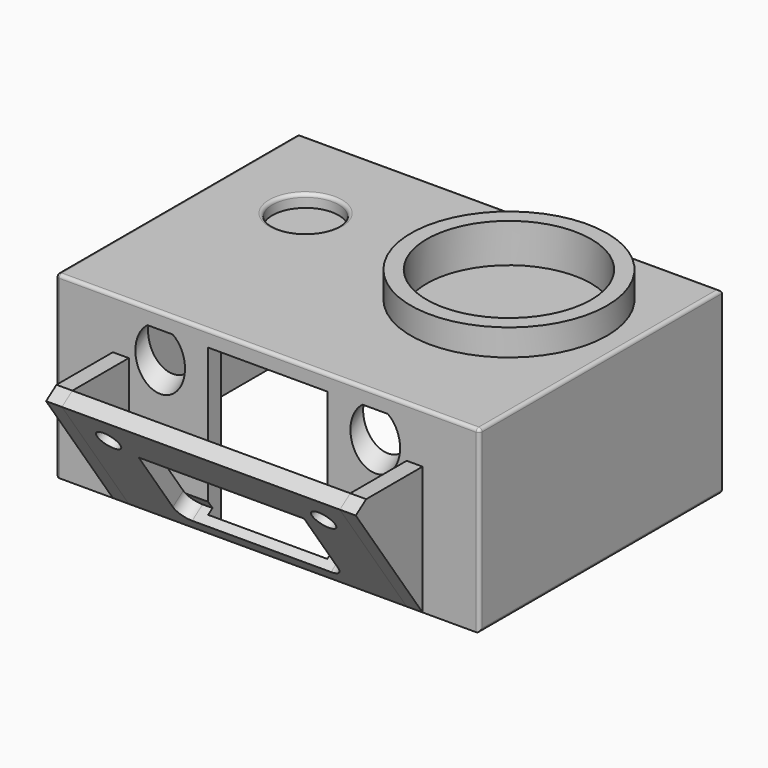
from build123d import *

# Parameters (mm, degrees)
F5_W         = 64
F5_H         = 45.8
F5_W_2       = 59.2
F5_H_2       = 41
F6_DEPTH     = 24.7
F7_W         = 64
F7_H         = 45.8
F7_W_2       = 59.2
F7_H_2       = 41
F8_DEPTH     = 2.4
F9_R         = 5
F10_DEPTH    = 1.9
F11_R        = 14.82
F11_R_2      = 12.42
F12_DEPTH    = 4
F13_DEPTH    = 1.9
F14_R        = 5
F15_DEPTH    = 2.4
F17_R        = 1.75
F18_DEPTH    = 2.4
F20_DEPTH    = 2.4
F22_DEPTH    = 2.4
F23_R        = 1.75
F24_REACH    = 60.3061382673
F25_R        = 0.5
F26_W        = 18
F26_H        = 2.4
F27_DEPTH    = 24.7
F28_R        = 3.75
F29_REACH    = 63.5629925168
F31_DEPTH    = 2.4
F32_T1_DEPTH = 2.4


# Not quite as in the source:
# - a fillet or chamfer that OpenCascade refuses, or shapes differently, is made with other operations: its cross-section is extruded or revolved along the edge and cut away or added
# - a feature names something its author has since deleted; it is built from what else it names


with BuildPart() as f6:
    # F5 (on Top) → F6 (new body)
    with BuildSketch(Plane.XY):
        Rectangle(F5_W, F5_H)
        Rectangle(F5_W_2, F5_H_2, mode=Mode.SUBTRACT)
    extrude(amount=F6_DEPTH)

    # F7 (on face) → F8 (join)
    with BuildSketch(Plane.XY.offset(24.7)):
        Rectangle(F7_W, F7_H)
        Rectangle(F7_W_2, F7_H_2, mode=Mode.SUBTRACT)
        Rectangle(F7_W_2, F7_H_2)
    extrude(amount=F8_DEPTH)

    # F9 (on face) → F10 (cut)
    with BuildSketch(Plane.XY.offset(27.1)):
        with Locations((-18.6, 7.5)):
            Circle(F9_R)
    extrude(amount=-F10_DEPTH, mode=Mode.SUBTRACT)

    # F11 (on face) → F12 (join)
    with BuildSketch(Plane.XY.offset(27.1)):
        with Locations((13.926, 5.264)):
            Circle(F11_R)
        with Locations((13.926, 5.264)):
            Circle(F11_R_2, mode=Mode.SUBTRACT)
    extrude(amount=F12_DEPTH)

    # F13 (cut): a face of the model
    f13_faces = [f6.faces().sort_by_distance(p)[0] for p in [
        (13.926, 5.264, 27.1),
    ]]
    extrude(f13_faces, amount=-F13_DEPTH, mode=Mode.SUBTRACT)

    # F14 (on face) → F15 (cut)
    with BuildSketch(Plane(origin=(0, 22.9, 0), x_dir=(-1, 0, 0), z_dir=(0, 1, 0))):
        with Locations((17.1, 13.55)):
            Circle(F14_R)
    extrude(amount=-F15_DEPTH, mode=Mode.SUBTRACT)

    # F17 (on face) → F18 (join)
    with BuildSketch(Plane(origin=(0, -15.3661306411, -10.759480508), x_dir=(-1, 0, 0), z_dir=(0, 0.8191520443, 0.5735764364))):
        Polygon((0, 24.1349003924), (0, 13.1349003924), (21, 13.1349003924), (21, 35.1349003924), (0, 35.1349003924), align=None)
        with Locations((16.25, 30.1349003924)):
            Circle(F17_R, mode=Mode.SUBTRACT)
        Polygon((-21, 13.1349003924), (0, 13.1349003924), (0, 24.1349003924), (0, 35.1349003924), (-21, 35.1349003924), align=None)
        with Locations((-16.25, 30.1349003924)):
            Circle(F17_R, mode=Mode.SUBTRACT)
    extrude(amount=F18_DEPTH)

    # F19 (on face) → F20 (join)
    with BuildSketch(Plane(origin=(-21, 0, 0), x_dir=(0, -1, 0), z_dir=(-1, 0, 0))):
        Polygon((22.9, 0), (35.5186815997, 18.0213449744), (33.5527166934, 19.3979284216), (22.9, 19.3979284216), align=None)
    extrude(amount=F20_DEPTH)

    # F21 (on face) → F22 (join)
    with BuildSketch(Plane.YZ.offset(21)):
        Polygon((-35.5186815997, 18.0213449744), (-22.9, 0), (-22.9, 19.3979284216), (-33.5527166934, 19.3979284216), align=None)
    extrude(amount=F22_DEPTH)

    f24_end = f6.faces().sort_by_distance((0, 0, 24.7))[0]
    # F23 (on face) → F24 (cut, up to a face of the model that its end follows)
    with BuildSketch(Plane(origin=(0, -15.3661306411, -10.759480508), x_dir=(1, 0, 0), z_dir=(0, -0.8191520443, -0.5735764364))):
        with Locations((-16.25, 30.1349003924)):
            Circle(F23_R)
        with Locations((16.25, 30.1349003924)):
            Circle(F23_R)
    f24_long = extrude(amount=-F24_REACH, mode=Mode.PRIVATE)
    add(split(f24_long, bisect_by=f24_end, keep=Keep.TOP, mode=Mode.PRIVATE), mode=Mode.SUBTRACT)

    # F25
    f25_edges = [f6.edges().sort_by_distance(p)[0] for p in [
        (-32, 0, 27.1),
        (0, -22.9, 27.1),
        (32, 0, 27.1),
        (0, 22.9, 27.1),
        (-23.6, 7.5, 27.1),
        (32, 0, 0),
        (0, 22.9, 0),
        (-32, 22.9, 13.55),
        (-32, 0, 0),
        (-32, -22.9, 13.55),
        (32, -22.9, 13.55),
    ]]
    fillet(f25_edges, radius=F25_R)

    # F26 (on face) → F27 (cut, through all)
    with BuildSketch(Plane(origin=(0, 0, 0), x_dir=(1, 0, 0), z_dir=(0, 0, -1))):
        with Locations((0, 21.7)):
            Rectangle(F26_W, F26_H)
    extrude(amount=-F27_DEPTH, mode=Mode.SUBTRACT)

    f29_end = Plane(origin=(0, -0.3794689119, 24.7), x_dir=(-1, 0, 0), z_dir=(0, 0, -1))
    # F28 (on face) → F29 (cut, up to a plane its end follows)
    with BuildSketch(Plane(origin=(0, -13.4001657348, -9.3828970608), x_dir=(-1, 0, 0), z_dir=(0, 0.8191520443, 0.5735764364))):
        with Locations((16.25, 30.1349003924)):
            Circle(F28_R)
        with Locations((-16.25, 30.1349003924)):
            Circle(F28_R)
    f29_long = extrude(amount=F29_REACH, mode=Mode.PRIVATE)
    add(split(f29_long, bisect_by=f29_end, keep=Keep.TOP, mode=Mode.PRIVATE), mode=Mode.SUBTRACT)

    # F30 (on face) → F31 (cut)
    with BuildSketch(Plane(origin=(0, -15.3661306411, -10.759480508), x_dir=(1, 0, 0), z_dir=(0, -0.8191520443, -0.5735764364))):
        Polygon((12.5, 28.3849003924), (-12.5, 28.3849003924), (-12.5, 15.1349003924), (0, 15.1349003924), (12.5, 15.1349003924), align=None)
    extrude(amount=-F31_DEPTH, mode=Mode.SUBTRACT)

    # F32: fillet of radius 2 on 2 edges, made by hand

    # F32_s2 → F32_t1 (join)
    with BuildSketch(Plane(origin=(0, -15.3661306411, -10.759480508), x_dir=(1, 0, 0), z_dir=(0, 0.8191520443, 0.5735764364))):
        with BuildLine():
            ThreePointArc((-10.5, -15.1349003924), (-11.9142135624, -15.7206868301), (-12.5, -17.1349003924))
            Line((-12.5, -17.1349003924), (-12.5, -15.1349003924))
            Line((-12.5, -15.1349003924), (-10.5, -15.1349003924))
        make_face()
        with BuildLine():
            ThreePointArc((12.5, -17.1349003924), (11.9142135624, -15.7206868301), (10.5, -15.1349003924))
            Line((10.5, -15.1349003924), (12.5, -15.1349003924))
            Line((12.5, -15.1349003924), (12.5, -17.1349003924))
        make_face()
    extrude(amount=F32_T1_DEPTH)


solid = f6.part
